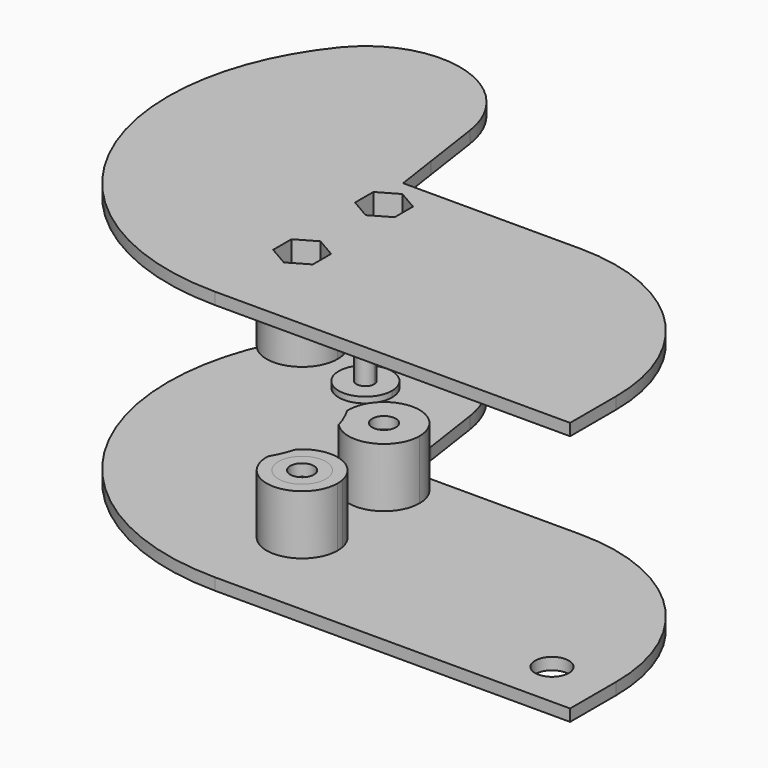
from build123d import *
from build123d import SkipClean  # not in build123d's __all__

# Parameters (mm, degrees)
F0_R      = 4
F1_DEPTH  = 2
F2_DEPTH  = 1
F3_DEPTH  = 10
F4_DEPTH  = 10
F5_R      = 4
F5_R_2    = 2
F6_DEPTH  = 2
F9_DEPTH  = 2
F10_DEPTH = 12
F11_R     = 6
F11_R_2   = 2
F12_DEPTH = 2
F13_DEPTH = 12
F14_R     = 30
F14_2_R   = 30
F15_R     = 2.85
F16_DEPTH = 2


# Not quite as in the source:
# - a feature names something its author has since deleted; it is built from what else it names


with BuildPart() as f1:
    # F0 (on Top) → F1 (new body)
    with BuildSketch(Plane.XY):
        with BuildLine():
            Line((58.100134976, 15), (42.100134976, 15))
            ThreePointArc((42.100134976, 15), (37.6910148186, 1.2250837024), (26.1026494547, -7.4293052282))
            ThreePointArc((26.1026494547, -7.4293052282), (26.1966821755, -8.0364360902), (26.2281363452, -8.65))
            ThreePointArc((26.2281363452, -8.65), (20.0819711782, -14.6482193811), (14.2352577639, -8.3577564209))
            ThreePointArc((14.2352577639, -8.3577564209), (14.2313656207, -8.3570657963), (14.2274735926, -8.3563745231))
            ThreePointArc((14.2274735926, -8.3563745231), (3.8773806963, -16.0379524546), (-8.8387484709, -13.9329295365))
            ThreePointArc((-8.8387484709, -13.9329295365), (3.7392709335, -21.9265497331), (18.3778670292, -24.7222679468))
            ThreePointArc((18.3778670292, -24.7222679468), (46.4657520585, -13.0878850293), (58.100134976, 15))
        make_face()
        with BuildLine():
            ThreePointArc((26.1026494547, -7.4293052282), (37.6910148186, 1.2250837024), (42.100134976, 15))
            Line((42.100134976, 15), (18.3778670292, 15))
            Line((18.3778670292, 15), (11.6619037897, 15))
            ThreePointArc((11.6619037897, 15), (10.5853788563, 14.2218583328), (9.4571172126, 13.5208333333))
            ThreePointArc((9.4571172126, 13.5208333333), (12.1263112553, 11.1893956646), (14.2360603918, 8.3417375001))
            ThreePointArc((14.2360603918, 8.3417375001), (20.0739541807, 14.6480186612), (26.2281363452, 8.65))
            ThreePointArc((26.2281363452, 8.65), (22.4446837804, 3.0744356817), (15.8658305227, 4.5304990701))
            ThreePointArc((15.8658305227, 4.5304990701), (16.3406885354, 2.2873342973), (16.5, 0))
            ThreePointArc((16.5, 0), (16.3406885354, -2.2873342973), (15.8658305227, -4.5304990701))
            ThreePointArc((15.8658305227, -4.5304990701), (21.8629029968, -2.876999221), (26.1026494547, -7.4293052282))
        make_face()
        with BuildLine():
            ThreePointArc((26.2281363452, -8.65), (26.1966821755, -8.0364360902), (26.1026494547, -7.4293052282))
            ThreePointArc((26.1026494547, -7.4293052282), (25.145129633, -7.7365378497), (24.1754492625, -8.0029136587))
            ThreePointArc((24.1754492625, -8.0029136587), (24.2149428159, -8.3253861287), (24.2281363452, -8.65))
            ThreePointArc((24.2281363452, -8.65), (20.2154709299, -12.6499799484), (16.2282165516, -8.6246692964))
            ThreePointArc((16.2282165516, -8.6246692964), (15.2289078696, -8.5123383089), (14.2352577639, -8.3577564209))
            ThreePointArc((14.2352577639, -8.3577564209), (20.0819711782, -14.6482193811), (26.2281363452, -8.65))
        make_face()
        with BuildLine():
            ThreePointArc((24.1754492625, -8.0029136587), (25.145129633, -7.7365378497), (26.1026494547, -7.4293052282))
            ThreePointArc((26.1026494547, -7.4293052282), (21.8629029968, -2.876999221), (15.8658305227, -4.5304990701))
            ThreePointArc((15.8658305227, -4.5304990701), (15.1711022589, -6.4875), (14.2360603918, -8.3417375001))
            ThreePointArc((14.2360603918, -8.3417375001), (14.2356537252, -8.3497466923), (14.2352577639, -8.3577564209))
            ThreePointArc((14.2352577639, -8.3577564209), (15.2289078696, -8.5123383089), (16.2282165516, -8.6246692964))
            ThreePointArc((16.2282165516, -8.6246692964), (19.916147741, -4.6621856725), (24.1754492625, -8.0029136587))
        make_face()
        with BuildLine():
            Line((11.6619037897, 15), (18.3778670292, 15))
            Line((18.3778670292, 15), (17.3205716767, 22.1898913713))
            ThreePointArc((17.3205716767, 22.1898913713), (14.9304924742, 18.2492385576), (11.6619037897, 15))
        make_face()
        with BuildLine():
            Line((78.3778670292, 15), (58.100134976, 15))
            ThreePointArc((58.100134976, 15), (46.4657520585, -13.0878850293), (18.3778670292, -24.7222679468))
            Line((18.3778670292, -24.7222679468), (78.3778670292, -24.7222679468))
            Line((78.3778670292, -24.7222679468), (78.3778670292, 15))
        make_face()
        with BuildLine():
            ThreePointArc((14.2360603918, -8.3417375001), (14.7113718874, -6.2909090909), (15.8658305227, -4.5304990701))
            ThreePointArc((15.8658305227, -4.5304990701), (16.3406885354, -2.2873342973), (16.5, 0))
            ThreePointArc((16.5, 0), (16.3406885354, 2.2873342973), (15.8658305227, 4.5304990701))
            ThreePointArc((15.8658305227, 4.5304990701), (14.7113718874, 6.2909090909), (14.2360603918, 8.3417375001))
            ThreePointArc((14.2360603918, 8.3417375001), (12.1263112553, 11.1893956646), (9.4571172126, 13.5208333333))
            ThreePointArc((9.4571172126, 13.5208333333), (2.354500942, 11.1464505911), (-5.113909886, 11.7011496077))
            ThreePointArc((-5.113909886, 11.7011496077), (1.3016126389, -1.4665580052), (14.2274735926, -8.3563745231))
            ThreePointArc((14.2274735926, -8.3563745231), (14.231768874, -8.3490571155), (14.2360603918, -8.3417375001))
        make_face()
        with BuildLine():
            ThreePointArc((14.2360603918, -8.3417375001), (15.1711022589, -6.4875), (15.8658305227, -4.5304990701))
            ThreePointArc((15.8658305227, -4.5304990701), (14.7113718874, -6.2909090909), (14.2360603918, -8.3417375001))
        make_face()
        with BuildLine():
            Line((6.8738635424, 15), (11.6619037897, 15))
            ThreePointArc((11.6619037897, 15), (14.9304924742, 18.2492385576), (17.3205716767, 22.1898913713))
            Line((17.3205716767, 22.1898913713), (15.8297593001, 32.3278145331))
            ThreePointArc((15.8297593001, 32.3278145331), (15.9573830687, 31.1670156808), (16, 30))
            ThreePointArc((16, 30), (13.3414037895, 21.1678459634), (6.2491318842, 15.2708333333))
            ThreePointArc((6.2491318842, 15.2708333333), (6.562894934, 15.1386396379), (6.8738635424, 15))
        make_face()
        with BuildLine():
            ThreePointArc((9.4571172126, 13.5208333333), (10.5853788563, 14.2218583328), (11.6619037897, 15))
            Line((11.6619037897, 15), (6.8738635424, 15))
            ThreePointArc((6.8738635424, 15), (8.1989155754, 14.3187912684), (9.4571172126, 13.5208333333))
        make_face()
        with BuildLine():
            ThreePointArc((15.8297593001, 32.3278145331), (15.0618472395, 35.3982180146), (13.7045776595, 38.2573937278))
            ThreePointArc((13.7045776595, 38.2573937278), (8.1175093349, 36.3885730362), (3.1632570293, 33.2005944709))
            ThreePointArc((3.1632570293, 33.2005944709), (4.1523882665, 31.734264018), (4.5, 30))
            ThreePointArc((4.5, 30), (2.1202896476, 26.0308222753), (-2.5019430268, 26.2596415826))
            ThreePointArc((-2.5019430268, 26.2596415826), (-4.5458381145, 21.1032564281), (-5.3364742263, 15.6132009157))
            ThreePointArc((-5.3364742263, 15.6132009157), (0.4873806423, 16.4928002507), (6.2491318842, 15.2708333333))
            ThreePointArc((6.2491318842, 15.2708333333), (13.3414037895, 21.1678459634), (16, 30))
            ThreePointArc((16, 30), (15.9573830687, 31.1670156808), (15.8297593001, 32.3278145331))
        make_face()
        with BuildLine():
            ThreePointArc((3.1632570293, 33.2005944709), (8.1175093349, 36.3885730362), (13.7045776595, 38.2573937278))
            ThreePointArc((13.7045776595, 38.2573937278), (1.1371555726, 45.9595387529), (-12.395352396, 40.1170766025))
            ThreePointArc((-12.395352396, 40.1170766025), (-15.5318430865, 26.1578846536), (-6.2491318842, 15.2708333333))
            ThreePointArc((-6.2491318842, 15.2708333333), (-5.7953318392, 15.4487581661), (-5.3364742263, 15.6132009157))
            ThreePointArc((-5.3364742263, 15.6132009157), (-4.5458381145, 21.1032564281), (-2.5019430268, 26.2596415826))
            ThreePointArc((-2.5019430268, 26.2596415826), (-3.4861928807, 32.8454277707), (3.1632570293, 33.2005944709))
        make_face()
        with BuildLine():
            ThreePointArc((-5.113909886, 11.7011496077), (2.354500942, 11.1464505911), (9.4571172126, 13.5208333333))
            ThreePointArc((9.4571172126, 13.5208333333), (8.1989155754, 14.3187912684), (6.8738635424, 15))
            Line((6.8738635424, 15), (5.5677643628, 15))
            ThreePointArc((5.5677643628, 15), (0.1188765047, 14.0004416193), (-5.3442623691, 14.9189237874))
            ThreePointArc((-5.3442623691, 14.9189237874), (-5.2838479343, 13.3061164355), (-5.113909886, 11.7011496077))
        make_face()
        with BuildLine():
            Line((5.5677643628, 15), (6.8738635424, 15))
            ThreePointArc((6.8738635424, 15), (6.562894934, 15.1386396379), (6.2491318842, 15.2708333333))
            ThreePointArc((6.2491318842, 15.2708333333), (5.9099997379, 15.1315130865), (5.5677643628, 15))
        make_face()
        with BuildLine():
            ThreePointArc((-15.4212723827, -5.8680795919), (-12.3953524648, -10.1170765181), (-8.8387484709, -13.9329295365))
            ThreePointArc((-8.8387484709, -13.9329295365), (3.8773806963, -16.0379524546), (14.2274735926, -8.3563745231))
            ThreePointArc((14.2274735926, -8.3563745231), (1.3016126389, -1.4665580052), (-5.113909886, 11.7011496077))
            ThreePointArc((-5.113909886, 11.7011496077), (-7.3421059576, 12.4759171393), (-9.4571172126, 13.5208333333))
            ThreePointArc((-9.4571172126, 13.5208333333), (-15.7707340768, 4.8511799266), (-15.4212723827, -5.8680795919))
        make_face()
        with BuildLine():
            ThreePointArc((4.5, 30), (4.1523882665, 31.734264018), (3.1632570293, 33.2005944709))
            ThreePointArc((3.1632570293, 33.2005944709), (2.0412089663, 32.2005697545), (0.9847414412, 31.1314964843))
            ThreePointArc((0.9847414412, 31.1314964843), (1.3651212697, 30.6216461366), (1.5, 30))
            ThreePointArc((1.5, 30), (0.6644948603, 28.655215043), (-0.9112621076, 28.8085297439))
            ThreePointArc((-0.9112621076, 28.8085297439), (-1.7469963662, 27.5592941625), (-2.5019430268, 26.2596415826))
            ThreePointArc((-2.5019430268, 26.2596415826), (2.1202896476, 26.0308222753), (4.5, 30))
        make_face()
        with BuildLine():
            ThreePointArc((0.9847414412, 31.1314964843), (2.0412089663, 32.2005697545), (3.1632570293, 33.2005944709))
            ThreePointArc((3.1632570293, 33.2005944709), (-3.4861928807, 32.8454277707), (-2.5019430268, 26.2596415826))
            ThreePointArc((-2.5019430268, 26.2596415826), (-1.7469963662, 27.5592941625), (-0.9112621076, 28.8085297439))
            ThreePointArc((-0.9112621076, 28.8085297439), (-1.1620642936, 30.9484759236), (0.9847414412, 31.1314964843))
        make_face()
        with BuildLine():
            ThreePointArc((-6.2491318842, 15.2708333333), (-15.5318430865, 26.1578846536), (-12.395352396, 40.1170766025))
            ThreePointArc((-12.395352396, 40.1170766025), (-16.1558630014, 34.6285521886), (-18.9475622454, 28.5893671785))
            ThreePointArc((-18.9475622454, 28.5893671785), (-16.745225523, 21.0223932931), (-11.6619037897, 15))
            Line((-11.6619037897, 15), (-6.8738635424, 15))
            ThreePointArc((-6.8738635424, 15), (-6.562894934, 15.1386396379), (-6.2491318842, 15.2708333333))
        make_face()
        with BuildLine():
            ThreePointArc((-11.6619037897, 15), (-16.745225523, 21.0223932931), (-18.9475622454, 28.5893671785))
            ThreePointArc((-18.9475622454, 28.5893671785), (-20.7406022259, 21.8995604195), (-21.3444009177, 15))
            Line((-21.3444009177, 15), (-11.6619037897, 15))
        make_face()
        with BuildLine():
            ThreePointArc((14.2360603918, 8.3417375001), (14.7113718874, 6.2909090909), (15.8658305227, 4.5304990701))
            ThreePointArc((15.8658305227, 4.5304990701), (15.1711022589, 6.4875), (14.2360603918, 8.3417375001))
        make_face()
        with BuildLine():
            ThreePointArc((14.2360603918, 8.3417375001), (15.1711022589, 6.4875), (15.8658305227, 4.5304990701))
            ThreePointArc((15.8658305227, 4.5304990701), (22.4446837804, 3.0744356817), (26.2281363452, 8.65))
            ThreePointArc((26.2281363452, 8.65), (20.0739541807, 14.6480186612), (14.2360603918, 8.3417375001))
        make_face()
        with Locations((20.2281363452, 8.65)):
            Circle(F0_R, mode=Mode.SUBTRACT)
        with BuildLine():
            ThreePointArc((-9.4571172126, 13.5208333333), (-7.3421059576, 12.4759171393), (-5.113909886, 11.7011496077))
            ThreePointArc((-5.113909886, 11.7011496077), (-5.2838479343, 13.3061164355), (-5.3442623691, 14.9189237874))
            ThreePointArc((-5.3442623691, 14.9189237874), (-5.4561639627, 14.9590467452), (-5.5677643628, 15))
            Line((-5.5677643628, 15), (-6.8738635424, 15))
            ThreePointArc((-6.8738635424, 15), (-8.1989155754, 14.3187912684), (-9.4571172126, 13.5208333333))
        make_face()
        with BuildLine():
            ThreePointArc((5.5677643628, 15), (5.9099997379, 15.1315130865), (6.2491318842, 15.2708333333))
            ThreePointArc((6.2491318842, 15.2708333333), (0.4873806423, 16.4928002507), (-5.3364742263, 15.6132009157))
            ThreePointArc((-5.3364742263, 15.6132009157), (-5.342419162, 15.3066260733), (-5.3444009177, 15))
            Line((-5.3444009177, 15), (5.5677643628, 15))
        make_face()
        with BuildLine():
            ThreePointArc((-5.3442623691, 14.9189237874), (0.1188765047, 14.0004416193), (5.5677643628, 15))
            Line((5.5677643628, 15), (-5.3444009177, 15))
            ThreePointArc((-5.3444009177, 15), (-5.3443662805, 14.9594618345), (-5.3442623691, 14.9189237874))
        make_face()
        with BuildLine():
            ThreePointArc((-21.3444009177, 15), (-19.834938697, 4.1538002335), (-15.4212723827, -5.8680795919))
            ThreePointArc((-15.4212723827, -5.8680795919), (-15.7707340768, 4.8511799266), (-9.4571172126, 13.5208333333))
            ThreePointArc((-9.4571172126, 13.5208333333), (-10.5853788563, 14.2218583328), (-11.6619037897, 15))
            Line((-11.6619037897, 15), (-21.3444009177, 15))
        make_face()
        with BuildLine():
            ThreePointArc((-5.5677643628, 15), (-5.9099997379, 15.1315130865), (-6.2491318842, 15.2708333333))
            ThreePointArc((-6.2491318842, 15.2708333333), (-6.562894934, 15.1386396379), (-6.8738635424, 15))
            Line((-6.8738635424, 15), (-5.5677643628, 15))
        make_face()
        with BuildLine():
            ThreePointArc((-5.3364742263, 15.6132009157), (-5.7953318392, 15.4487581661), (-6.2491318842, 15.2708333333))
            ThreePointArc((-6.2491318842, 15.2708333333), (-5.9099997379, 15.1315130865), (-5.5677643628, 15))
            Line((-5.5677643628, 15), (-5.3444009177, 15))
            ThreePointArc((-5.3444009177, 15), (-5.342419162, 15.3066260733), (-5.3364742263, 15.6132009157))
        make_face()
        with BuildLine():
            Line((-6.8738635424, 15), (-11.6619037897, 15))
            ThreePointArc((-11.6619037897, 15), (-10.5853788563, 14.2218583328), (-9.4571172126, 13.5208333333))
            ThreePointArc((-9.4571172126, 13.5208333333), (-8.1989155754, 14.3187912684), (-6.8738635424, 15))
        make_face()
        with BuildLine():
            ThreePointArc((-5.5677643628, 15), (-5.4561639627, 14.9590467452), (-5.3442623691, 14.9189237874))
            ThreePointArc((-5.3442623691, 14.9189237874), (-5.3443662805, 14.9594618345), (-5.3444009177, 15))
            Line((-5.3444009177, 15), (-5.5677643628, 15))
        make_face()
    extrude(amount=-F1_DEPTH)

    # F0 (on Top) → F2 (join)
    with BuildSketch(Plane.XY):
        with BuildLine():
            ThreePointArc((4.5, 30), (4.1523882665, 31.734264018), (3.1632570293, 33.2005944709))
            ThreePointArc((3.1632570293, 33.2005944709), (2.0412089663, 32.2005697545), (0.9847414412, 31.1314964843))
            ThreePointArc((0.9847414412, 31.1314964843), (1.3651212697, 30.6216461366), (1.5, 30))
            ThreePointArc((1.5, 30), (0.6644948603, 28.655215043), (-0.9112621076, 28.8085297439))
            ThreePointArc((-0.9112621076, 28.8085297439), (-1.7469963662, 27.5592941625), (-2.5019430268, 26.2596415826))
            ThreePointArc((-2.5019430268, 26.2596415826), (2.1202896476, 26.0308222753), (4.5, 30))
        make_face()
        with BuildLine():
            ThreePointArc((0.9847414412, 31.1314964843), (2.0412089663, 32.2005697545), (3.1632570293, 33.2005944709))
            ThreePointArc((3.1632570293, 33.2005944709), (-3.4861928807, 32.8454277707), (-2.5019430268, 26.2596415826))
            ThreePointArc((-2.5019430268, 26.2596415826), (-1.7469963662, 27.5592941625), (-0.9112621076, 28.8085297439))
            ThreePointArc((-0.9112621076, 28.8085297439), (-1.1620642936, 30.9484759236), (0.9847414412, 31.1314964843))
        make_face()
    with SkipClean():  # cleaning this boolean's faces spoils the solid; the shape is the same uncleaned
        extrude(amount=F2_DEPTH)

    # F0 (on Top) → F3 (join)
    with BuildSketch(Plane.XY):
        with BuildLine():
            ThreePointArc((1.5, 30), (1.3651212697, 30.6216461366), (0.9847414412, 31.1314964843))
            ThreePointArc((0.9847414412, 31.1314964843), (0, 30), (-0.9112621076, 28.8085297439))
            ThreePointArc((-0.9112621076, 28.8085297439), (0.6644948603, 28.655215043), (1.5, 30))
        make_face()
        with BuildLine():
            ThreePointArc((-0.9112621076, 28.8085297439), (0, 30), (0.9847414412, 31.1314964843))
            ThreePointArc((0.9847414412, 31.1314964843), (-1.1620642936, 30.9484759236), (-0.9112621076, 28.8085297439))
        make_face()
    extrude(amount=F3_DEPTH)

    # F0 (on Top) → F4 (join)
    with BuildSketch(Plane.XY):
        with BuildLine():
            ThreePointArc((26.2281363452, -8.65), (26.1966821755, -8.0364360902), (26.1026494547, -7.4293052282))
            ThreePointArc((26.1026494547, -7.4293052282), (25.145129633, -7.7365378497), (24.1754492625, -8.0029136587))
            ThreePointArc((24.1754492625, -8.0029136587), (24.2149428159, -8.3253861287), (24.2281363452, -8.65))
            ThreePointArc((24.2281363452, -8.65), (20.2154709299, -12.6499799484), (16.2282165516, -8.6246692964))
            ThreePointArc((16.2282165516, -8.6246692964), (15.2289078696, -8.5123383089), (14.2352577639, -8.3577564209))
            ThreePointArc((14.2352577639, -8.3577564209), (20.0819711782, -14.6482193811), (26.2281363452, -8.65))
        make_face()
        with BuildLine():
            ThreePointArc((14.2360603918, 8.3417375001), (15.1711022589, 6.4875), (15.8658305227, 4.5304990701))
            ThreePointArc((15.8658305227, 4.5304990701), (22.4446837804, 3.0744356817), (26.2281363452, 8.65))
            ThreePointArc((26.2281363452, 8.65), (20.0739541807, 14.6480186612), (14.2360603918, 8.3417375001))
        make_face()
        with Locations((20.2281363452, 8.65)):
            Circle(F0_R, mode=Mode.SUBTRACT)
        with BuildLine():
            ThreePointArc((24.1754492625, -8.0029136587), (25.145129633, -7.7365378497), (26.1026494547, -7.4293052282))
            ThreePointArc((26.1026494547, -7.4293052282), (21.8629029968, -2.876999221), (15.8658305227, -4.5304990701))
            ThreePointArc((15.8658305227, -4.5304990701), (15.1711022589, -6.4875), (14.2360603918, -8.3417375001))
            ThreePointArc((14.2360603918, -8.3417375001), (14.2356537252, -8.3497466923), (14.2352577639, -8.3577564209))
            ThreePointArc((14.2352577639, -8.3577564209), (15.2289078696, -8.5123383089), (16.2282165516, -8.6246692964))
            ThreePointArc((16.2282165516, -8.6246692964), (19.916147741, -4.6621856725), (24.1754492625, -8.0029136587))
        make_face()
    extrude(amount=F4_DEPTH)

    # F5 (on face) → F6 (join)
    with BuildSketch(Plane.XY.offset(10)):
        with Locations((20.2281363452, 8.65)):
            Circle(F5_R)
        with Locations((20.2281363452, 8.65)):
            Circle(F5_R_2, mode=Mode.SUBTRACT)
        with Locations((20.2281363452, -8.65)):
            Circle(F5_R)
        with Locations((20.2281363452, -8.65)):
            Circle(F5_R_2, mode=Mode.SUBTRACT)
    extrude(amount=-F6_DEPTH)

    # F14
    f14_edges = [f1.edges().sort_by_distance(p)[0] for p in [
        (78.377867, 15, -1),
    ]]
    fillet(f14_edges, radius=F14_R)

    # F15 (on face) → F16 (cut, through all)
    with BuildSketch(Plane(origin=(0, 0, -2), x_dir=(1, 0, 0), z_dir=(0, 0, -1))):
        with Locations((69.0778670292, 16.9222679468)):
            Circle(F15_R)
    extrude(amount=-F16_DEPTH, mode=Mode.SUBTRACT)


with BuildPart() as f9:
    # F8 (on offset) → F9 (new body)
    with BuildSketch(Plane.XY.offset(40.5)):
        with BuildLine():
            Line((58.100134976, 15), (42.100134976, 15))
            ThreePointArc((42.100134976, 15), (37.6910148186, 1.2250837024), (26.1026494547, -7.4293052282))
            ThreePointArc((26.1026494547, -7.4293052282), (26.1966821755, -8.0364360902), (26.2281363452, -8.65))
            ThreePointArc((26.2281363452, -8.65), (20.0819711782, -14.6482193811), (14.2352577639, -8.3577564209))
            ThreePointArc((14.2352577639, -8.3577564209), (14.2313656207, -8.3570657963), (14.2274735926, -8.3563745231))
            ThreePointArc((14.2274735926, -8.3563745231), (3.8773806963, -16.0379524546), (-8.8387484709, -13.9329295365))
            ThreePointArc((-8.8387484709, -13.9329295365), (3.7392709335, -21.9265497331), (18.3778670292, -24.7222679468))
            ThreePointArc((18.3778670292, -24.7222679468), (46.4657520585, -13.0878850293), (58.100134976, 15))
        make_face()
        with BuildLine():
            ThreePointArc((26.1026494547, -7.4293052282), (37.6910148186, 1.2250837024), (42.100134976, 15))
            Line((42.100134976, 15), (18.3778670292, 15))
            Line((18.3778670292, 15), (11.6619037897, 15))
            ThreePointArc((11.6619037897, 15), (10.5853788563, 14.2218583328), (9.4571172126, 13.5208333333))
            ThreePointArc((9.4571172126, 13.5208333333), (12.1263112553, 11.1893956646), (14.2360603918, 8.3417375001))
            ThreePointArc((14.2360603918, 8.3417375001), (20.0739541807, 14.6480186612), (26.2281363452, 8.65))
            ThreePointArc((26.2281363452, 8.65), (22.4446837804, 3.0744356817), (15.8658305227, 4.5304990701))
            ThreePointArc((15.8658305227, 4.5304990701), (16.3406885354, 2.2873342973), (16.5, 0))
            ThreePointArc((16.5, 0), (16.3406885354, -2.2873342973), (15.8658305227, -4.5304990701))
            ThreePointArc((15.8658305227, -4.5304990701), (21.8629029968, -2.876999221), (26.1026494547, -7.4293052282))
        make_face()
        with BuildLine():
            ThreePointArc((26.2281363452, -8.65), (26.1966821755, -8.0364360902), (26.1026494547, -7.4293052282))
            ThreePointArc((26.1026494547, -7.4293052282), (24.8503000713, -7.8222174001), (23.5781363452, -8.1452629188))
            Line((23.5781363452, -8.1452629188), (23.5781363452, -10.5841234018))
            Line((23.5781363452, -10.5841234018), (20.2281363452, -12.5182468036))
            Line((20.2281363452, -12.5182468036), (16.8781363452, -10.5841234018))
            Line((16.8781363452, -10.5841234018), (16.8781363452, -8.6748137145))
            ThreePointArc((16.8781363452, -8.6748137145), (15.5522465031, -8.5533833065), (14.2352577639, -8.3577564209))
            ThreePointArc((14.2352577639, -8.3577564209), (20.0819711782, -14.6482193811), (26.2281363452, -8.65))
        make_face()
        with BuildLine():
            ThreePointArc((23.5781363452, -8.1452629188), (24.8503000713, -7.8222174001), (26.1026494547, -7.4293052282))
            ThreePointArc((26.1026494547, -7.4293052282), (21.8629029968, -2.876999221), (15.8658305227, -4.5304990701))
            ThreePointArc((15.8658305227, -4.5304990701), (15.1711022589, -6.4875), (14.2360603918, -8.3417375001))
            ThreePointArc((14.2360603918, -8.3417375001), (14.2356537252, -8.3497466923), (14.2352577639, -8.3577564209))
            ThreePointArc((14.2352577639, -8.3577564209), (15.5522465031, -8.5533833065), (16.8781363452, -8.6748137145))
            Line((16.8781363452, -8.6748137145), (16.8781363452, -6.7158765982))
            Line((16.8781363452, -6.7158765982), (20.2281363452, -4.7817531964))
            Line((20.2281363452, -4.7817531964), (23.5781363452, -6.7158765982))
            Line((23.5781363452, -6.7158765982), (23.5781363452, -8.1452629188))
        make_face()
        with BuildLine():
            Line((11.6619037897, 15), (18.3778670292, 15))
            Line((18.3778670292, 15), (17.3205716767, 22.1898913713))
            ThreePointArc((17.3205716767, 22.1898913713), (14.9304924742, 18.2492385576), (11.6619037897, 15))
        make_face()
        with BuildLine():
            Line((78.3778670292, 15), (58.100134976, 15))
            ThreePointArc((58.100134976, 15), (46.4657520585, -13.0878850293), (18.3778670292, -24.7222679468))
            Line((18.3778670292, -24.7222679468), (78.3778670292, -24.7222679468))
            Line((78.3778670292, -24.7222679468), (78.3778670292, 15))
        make_face()
        with BuildLine():
            ThreePointArc((14.2360603918, -8.3417375001), (14.7113718874, -6.2909090909), (15.8658305227, -4.5304990701))
            ThreePointArc((15.8658305227, -4.5304990701), (16.3406885354, -2.2873342973), (16.5, 0))
            ThreePointArc((16.5, 0), (16.3406885354, 2.2873342973), (15.8658305227, 4.5304990701))
            ThreePointArc((15.8658305227, 4.5304990701), (14.7113718874, 6.2909090909), (14.2360603918, 8.3417375001))
            ThreePointArc((14.2360603918, 8.3417375001), (12.1263112553, 11.1893956646), (9.4571172126, 13.5208333333))
            ThreePointArc((9.4571172126, 13.5208333333), (2.354500942, 11.1464505911), (-5.113909886, 11.7011496077))
            ThreePointArc((-5.113909886, 11.7011496077), (1.3016126389, -1.4665580052), (14.2274735926, -8.3563745231))
            ThreePointArc((14.2274735926, -8.3563745231), (14.231768874, -8.3490571155), (14.2360603918, -8.3417375001))
        make_face()
        with BuildLine():
            ThreePointArc((14.2360603918, -8.3417375001), (15.1711022589, -6.4875), (15.8658305227, -4.5304990701))
            ThreePointArc((15.8658305227, -4.5304990701), (14.7113718874, -6.2909090909), (14.2360603918, -8.3417375001))
        make_face()
        with BuildLine():
            Line((6.8738635424, 15), (11.6619037897, 15))
            ThreePointArc((11.6619037897, 15), (14.9304924742, 18.2492385576), (17.3205716767, 22.1898913713))
            Line((17.3205716767, 22.1898913713), (15.8297593556, 32.3278141558))
            ThreePointArc((15.8297593556, 32.3278141558), (15.9573830826, 31.1670154906), (16, 30))
            ThreePointArc((16, 30), (13.3414037895, 21.1678459634), (6.2491318842, 15.2708333333))
            ThreePointArc((6.2491318842, 15.2708333333), (6.562894934, 15.1386396379), (6.8738635424, 15))
        make_face()
        with BuildLine():
            ThreePointArc((9.4571172126, 13.5208333333), (10.5853788563, 14.2218583328), (11.6619037897, 15))
            Line((11.6619037897, 15), (6.8738635424, 15))
            ThreePointArc((6.8738635424, 15), (8.1989155754, 14.3187912684), (9.4571172126, 13.5208333333))
        make_face()
        with BuildLine():
            ThreePointArc((15.8297593556, 32.3278141558), (15.0618473039, 35.3982178351), (13.7045776595, 38.2573937278))
            ThreePointArc((13.7045776595, 38.2573937278), (7.8917709447, 36.2788107151), (2.781523926, 32.8745651234))
            ThreePointArc((2.781523926, 32.8745651234), (3.6828043462, 31.5610740366), (4, 30))
            ThreePointArc((4, 30), (1.8660095282, 26.4619202326), (-2.2590042204, 26.6989547213))
            ThreePointArc((-2.2590042204, 26.6989547213), (-4.4799761986, 21.3454707876), (-5.3364742263, 15.6132009157))
            ThreePointArc((-5.3364742263, 15.6132009157), (0.4873806423, 16.4928002507), (6.2491318842, 15.2708333333))
            ThreePointArc((6.2491318842, 15.2708333333), (13.3414037895, 21.1678459634), (16, 30))
            ThreePointArc((16, 30), (15.9573830826, 31.1670154906), (15.8297593556, 32.3278141558))
        make_face()
        with BuildLine():
            ThreePointArc((2.781523926, 32.8745651234), (7.8917709447, 36.2788107151), (13.7045776595, 38.2573937278))
            ThreePointArc((13.7045776595, 38.2573937278), (1.1371555726, 45.9595387529), (-12.395352396, 40.1170766025))
            ThreePointArc((-12.395352396, 40.1170766025), (-15.5318430865, 26.1578846536), (-6.2491318842, 15.2708333333))
            ThreePointArc((-6.2491318842, 15.2708333333), (-5.7953318392, 15.4487581661), (-5.3364742263, 15.6132009157))
            ThreePointArc((-5.3364742263, 15.6132009157), (-4.4799761986, 21.3454707876), (-2.2590042204, 26.6989547213))
            ThreePointArc((-2.2590042204, 26.6989547213), (-3.0988381162, 32.5292691295), (2.781523926, 32.8745651234))
        make_face()
        with BuildLine():
            ThreePointArc((14.2274735926, -8.3563745231), (14.2313656207, -8.3570657963), (14.2352577639, -8.3577564209))
            ThreePointArc((14.2352577639, -8.3577564209), (14.2356537252, -8.3497466923), (14.2360603918, -8.3417375001))
            ThreePointArc((14.2360603918, -8.3417375001), (14.231768874, -8.3490571155), (14.2274735926, -8.3563745231))
        make_face()
        with BuildLine():
            ThreePointArc((-5.113909886, 11.7011496077), (2.354500942, 11.1464505911), (9.4571172126, 13.5208333333))
            ThreePointArc((9.4571172126, 13.5208333333), (8.1989155754, 14.3187912684), (6.8738635424, 15))
            Line((6.8738635424, 15), (5.5677643628, 15))
            ThreePointArc((5.5677643628, 15), (0.1188765047, 14.0004416193), (-5.3442623691, 14.9189237874))
            ThreePointArc((-5.3442623691, 14.9189237874), (-5.2838479343, 13.3061164355), (-5.113909886, 11.7011496077))
        make_face()
        with BuildLine():
            Line((5.5677643628, 15), (6.8738635424, 15))
            ThreePointArc((6.8738635424, 15), (6.562894934, 15.1386396379), (6.2491318842, 15.2708333333))
            ThreePointArc((6.2491318842, 15.2708333333), (5.9099997379, 15.1315130865), (5.5677643628, 15))
        make_face()
        with BuildLine():
            ThreePointArc((-15.4212723827, -5.8680795919), (-12.3953524648, -10.1170765181), (-8.8387484709, -13.9329295365))
            ThreePointArc((-8.8387484709, -13.9329295365), (3.8773806963, -16.0379524546), (14.2274735926, -8.3563745231))
            ThreePointArc((14.2274735926, -8.3563745231), (1.3016126389, -1.4665580052), (-5.113909886, 11.7011496077))
            ThreePointArc((-5.113909886, 11.7011496077), (-7.3421059576, 12.4759171393), (-9.4571172126, 13.5208333333))
            ThreePointArc((-9.4571172126, 13.5208333333), (-15.7707340768, 4.8511799266), (-15.4212723827, -5.8680795919))
        make_face()
        with BuildLine():
            ThreePointArc((4, 30), (3.6828043462, 31.5610740366), (2.781523926, 32.8745651234))
            ThreePointArc((2.781523926, 32.8745651234), (2.0406007003, 32.1999920186), (1.3288254001, 31.4947317672))
            ThreePointArc((1.3288254001, 31.4947317672), (1.8245068923, 30.8192524641), (2, 30))
            ThreePointArc((2, 30), (0.8954353836, 28.2116500696), (-1.1981954737, 28.3986481939))
            ThreePointArc((-1.1981954737, 28.3986481939), (-1.7465522102, 27.5600058448), (-2.2590042204, 26.6989547213))
            ThreePointArc((-2.2590042204, 26.6989547213), (1.8660095282, 26.4619202326), (4, 30))
        make_face()
        with BuildLine():
            ThreePointArc((1.3288254001, 31.4947317672), (2.0406007003, 32.1999920186), (2.781523926, 32.8745651234))
            ThreePointArc((2.781523926, 32.8745651234), (-3.0988381162, 32.5292691295), (-2.2590042204, 26.6989547213))
            ThreePointArc((-2.2590042204, 26.6989547213), (-1.7465522102, 27.5600058448), (-1.1981954737, 28.3986481939))
            ThreePointArc((-1.1981954737, 28.3986481939), (-1.5494190581, 31.2646345648), (1.3288254001, 31.4947317672))
        make_face()
        with BuildLine():
            ThreePointArc((-6.2491318842, 15.2708333333), (-15.5318430865, 26.1578846536), (-12.395352396, 40.1170766025))
            ThreePointArc((-12.395352396, 40.1170766025), (-16.1558630014, 34.6285521886), (-18.9475622454, 28.5893671785))
            ThreePointArc((-18.9475622454, 28.5893671785), (-16.745225523, 21.0223932931), (-11.6619037897, 15))
            Line((-11.6619037897, 15), (-6.8738635424, 15))
            ThreePointArc((-6.8738635424, 15), (-6.562894934, 15.1386396379), (-6.2491318842, 15.2708333333))
        make_face()
        with BuildLine():
            ThreePointArc((-11.6619037897, 15), (-16.745225523, 21.0223932931), (-18.9475622454, 28.5893671785))
            ThreePointArc((-18.9475622454, 28.5893671785), (-20.7406022259, 21.8995604195), (-21.3444009177, 15))
            Line((-21.3444009177, 15), (-11.6619037897, 15))
        make_face()
        with BuildLine():
            ThreePointArc((14.2360603918, 8.3417375001), (14.7113718874, 6.2909090909), (15.8658305227, 4.5304990701))
            ThreePointArc((15.8658305227, 4.5304990701), (15.1711022589, 6.4875), (14.2360603918, 8.3417375001))
        make_face()
        with BuildLine():
            ThreePointArc((14.2360603918, 8.3417375001), (15.1711022589, 6.4875), (15.8658305227, 4.5304990701))
            ThreePointArc((15.8658305227, 4.5304990701), (22.4446837804, 3.0744356817), (26.2281363452, 8.65))
            ThreePointArc((26.2281363452, 8.65), (20.0739541807, 14.6480186612), (14.2360603918, 8.3417375001))
        make_face()
        Polygon((20.2281363452, 12.5182468036), (23.5781363452, 10.5841234018), (23.5781363452, 6.7158765982), (20.2281363452, 4.7817531964), (16.8781363452, 6.7158765982), (16.8781363452, 10.5841234018), align=None, mode=Mode.SUBTRACT)
        with BuildLine():
            ThreePointArc((-9.4571172126, 13.5208333333), (-7.3421059576, 12.4759171393), (-5.113909886, 11.7011496077))
            ThreePointArc((-5.113909886, 11.7011496077), (-5.2838479343, 13.3061164355), (-5.3442623691, 14.9189237874))
            ThreePointArc((-5.3442623691, 14.9189237874), (-5.4561639627, 14.9590467452), (-5.5677643628, 15))
            Line((-5.5677643628, 15), (-6.8738635424, 15))
            ThreePointArc((-6.8738635424, 15), (-8.1989155754, 14.3187912684), (-9.4571172126, 13.5208333333))
        make_face()
        with BuildLine():
            ThreePointArc((5.5677643628, 15), (5.9099997379, 15.1315130865), (6.2491318842, 15.2708333333))
            ThreePointArc((6.2491318842, 15.2708333333), (0.4873806423, 16.4928002507), (-5.3364742263, 15.6132009157))
            ThreePointArc((-5.3364742263, 15.6132009157), (-5.342419162, 15.3066260733), (-5.3444009177, 15))
            Line((-5.3444009177, 15), (5.5677643628, 15))
        make_face()
        with BuildLine():
            ThreePointArc((-5.3442623691, 14.9189237874), (0.1188765047, 14.0004416193), (5.5677643628, 15))
            Line((5.5677643628, 15), (-5.3444009177, 15))
            ThreePointArc((-5.3444009177, 15), (-5.3443662805, 14.9594618345), (-5.3442623691, 14.9189237874))
        make_face()
        with BuildLine():
            ThreePointArc((-21.3444009177, 15), (-19.834938697, 4.1538002335), (-15.4212723827, -5.8680795919))
            ThreePointArc((-15.4212723827, -5.8680795919), (-15.7707340768, 4.8511799266), (-9.4571172126, 13.5208333333))
            ThreePointArc((-9.4571172126, 13.5208333333), (-10.5853788563, 14.2218583328), (-11.6619037897, 15))
            Line((-11.6619037897, 15), (-21.3444009177, 15))
        make_face()
        with BuildLine():
            ThreePointArc((2, 30), (1.8245068923, 30.8192524641), (1.3288254001, 31.4947317672))
            ThreePointArc((1.3288254001, 31.4947317672), (0, 30), (-1.1981954737, 28.3986481939))
            ThreePointArc((-1.1981954737, 28.3986481939), (0.8954353836, 28.2116500696), (2, 30))
        make_face()
        with BuildLine():
            ThreePointArc((-1.1981954737, 28.3986481939), (0, 30), (1.3288254001, 31.4947317672))
            ThreePointArc((1.3288254001, 31.4947317672), (-1.5494190581, 31.2646345648), (-1.1981954737, 28.3986481939))
        make_face()
        with BuildLine():
            ThreePointArc((-5.5677643628, 15), (-5.9099997379, 15.1315130865), (-6.2491318842, 15.2708333333))
            ThreePointArc((-6.2491318842, 15.2708333333), (-6.562894934, 15.1386396379), (-6.8738635424, 15))
            Line((-6.8738635424, 15), (-5.5677643628, 15))
        make_face()
        with BuildLine():
            ThreePointArc((-5.3364742263, 15.6132009157), (-5.7953318392, 15.4487581661), (-6.2491318842, 15.2708333333))
            ThreePointArc((-6.2491318842, 15.2708333333), (-5.9099997379, 15.1315130865), (-5.5677643628, 15))
            Line((-5.5677643628, 15), (-5.3444009177, 15))
            ThreePointArc((-5.3444009177, 15), (-5.342419162, 15.3066260733), (-5.3364742263, 15.6132009157))
        make_face()
        with BuildLine():
            Line((-6.8738635424, 15), (-11.6619037897, 15))
            ThreePointArc((-11.6619037897, 15), (-10.5853788563, 14.2218583328), (-9.4571172126, 13.5208333333))
            ThreePointArc((-9.4571172126, 13.5208333333), (-8.1989155754, 14.3187912684), (-6.8738635424, 15))
        make_face()
        with BuildLine():
            ThreePointArc((-5.5677643628, 15), (-5.4561639627, 14.9590467452), (-5.3442623691, 14.9189237874))
            ThreePointArc((-5.3442623691, 14.9189237874), (-5.3443662805, 14.9594618345), (-5.3444009177, 15))
            Line((-5.3444009177, 15), (-5.5677643628, 15))
        make_face()
    extrude(amount=F9_DEPTH)

    # F8 (on offset) → F10 (join)
    with BuildSketch(Plane.XY.offset(40.5)):
        with BuildLine():
            ThreePointArc((26.2281363452, -8.65), (26.1966821755, -8.0364360902), (26.1026494547, -7.4293052282))
            ThreePointArc((26.1026494547, -7.4293052282), (24.8503000713, -7.8222174001), (23.5781363452, -8.1452629188))
            Line((23.5781363452, -8.1452629188), (23.5781363452, -10.5841234018))
            Line((23.5781363452, -10.5841234018), (20.2281363452, -12.5182468036))
            Line((20.2281363452, -12.5182468036), (16.8781363452, -10.5841234018))
            Line((16.8781363452, -10.5841234018), (16.8781363452, -8.6748137145))
            ThreePointArc((16.8781363452, -8.6748137145), (15.5522465031, -8.5533833065), (14.2352577639, -8.3577564209))
            ThreePointArc((14.2352577639, -8.3577564209), (20.0819711782, -14.6482193811), (26.2281363452, -8.65))
        make_face()
        with BuildLine():
            ThreePointArc((23.5781363452, -8.1452629188), (24.8503000713, -7.8222174001), (26.1026494547, -7.4293052282))
            ThreePointArc((26.1026494547, -7.4293052282), (21.8629029968, -2.876999221), (15.8658305227, -4.5304990701))
            ThreePointArc((15.8658305227, -4.5304990701), (15.1711022589, -6.4875), (14.2360603918, -8.3417375001))
            ThreePointArc((14.2360603918, -8.3417375001), (14.2356537252, -8.3497466923), (14.2352577639, -8.3577564209))
            ThreePointArc((14.2352577639, -8.3577564209), (15.5522465031, -8.5533833065), (16.8781363452, -8.6748137145))
            Line((16.8781363452, -8.6748137145), (16.8781363452, -6.7158765982))
            Line((16.8781363452, -6.7158765982), (20.2281363452, -4.7817531964))
            Line((20.2281363452, -4.7817531964), (23.5781363452, -6.7158765982))
            Line((23.5781363452, -6.7158765982), (23.5781363452, -8.1452629188))
        make_face()
        with BuildLine():
            ThreePointArc((14.2360603918, -8.3417375001), (15.1711022589, -6.4875), (15.8658305227, -4.5304990701))
            ThreePointArc((15.8658305227, -4.5304990701), (14.7113718874, -6.2909090909), (14.2360603918, -8.3417375001))
        make_face()
        with BuildLine():
            ThreePointArc((14.2360603918, 8.3417375001), (14.7113718874, 6.2909090909), (15.8658305227, 4.5304990701))
            ThreePointArc((15.8658305227, 4.5304990701), (15.1711022589, 6.4875), (14.2360603918, 8.3417375001))
        make_face()
        with BuildLine():
            ThreePointArc((14.2360603918, 8.3417375001), (15.1711022589, 6.4875), (15.8658305227, 4.5304990701))
            ThreePointArc((15.8658305227, 4.5304990701), (22.4446837804, 3.0744356817), (26.2281363452, 8.65))
            ThreePointArc((26.2281363452, 8.65), (20.0739541807, 14.6480186612), (14.2360603918, 8.3417375001))
        make_face()
        Polygon((20.2281363452, 12.5182468036), (23.5781363452, 10.5841234018), (23.5781363452, 6.7158765982), (20.2281363452, 4.7817531964), (16.8781363452, 6.7158765982), (16.8781363452, 10.5841234018), align=None, mode=Mode.SUBTRACT)
    extrude(amount=-F10_DEPTH)

    # F11 (on face) → F12 (join)
    with BuildSketch(Plane(origin=(0, 0, 28.5), x_dir=(1, 0, 0), z_dir=(0, 0, -1))):
        with Locations((20.2281363452, 8.65)):
            Circle(F11_R)
        Polygon((16.8781363452, 10.5841234018), (20.2281363452, 12.5182468036), (23.5781363452, 10.5841234018), (23.5781363452, 6.7158765982), (20.2281363452, 4.7817531964), (16.8781363452, 6.7158765982), align=None, mode=Mode.SUBTRACT)
        with Locations((20.2281363452, -8.65)):
            Circle(F11_R)
        with Locations((20.2281363452, -8.65)):
            Circle(F11_R_2, mode=Mode.SUBTRACT)
        Polygon((23.5781363452, 10.5841234018), (20.2281363452, 12.5182468036), (16.8781363452, 10.5841234018), (16.8781363452, 6.7158765982), (20.2281363452, 4.7817531964), (23.5781363452, 6.7158765982), align=None)
        with Locations((20.2281363452, 8.65)):
            Circle(F11_R_2, mode=Mode.SUBTRACT)
    extrude(amount=-F12_DEPTH)

    # F8 (on offset) → F13 (join)
    with BuildSketch(Plane.XY.offset(40.5)):
        with BuildLine():
            ThreePointArc((-1.1981954737, 28.3986481939), (0, 30), (1.3288254001, 31.4947317672))
            ThreePointArc((1.3288254001, 31.4947317672), (-1.5494190581, 31.2646345648), (-1.1981954737, 28.3986481939))
        make_face()
        with BuildLine():
            ThreePointArc((2, 30), (1.8245068923, 30.8192524641), (1.3288254001, 31.4947317672))
            ThreePointArc((1.3288254001, 31.4947317672), (0, 30), (-1.1981954737, 28.3986481939))
            ThreePointArc((-1.1981954737, 28.3986481939), (0.8954353836, 28.2116500696), (2, 30))
        make_face()
    extrude(amount=-F13_DEPTH)

    # F14#2
    f14_2_edges = [f9.edges().sort_by_distance(p)[0] for p in [
        (78.377867, 15, 41.5),
    ]]
    fillet(f14_2_edges, radius=F14_2_R)


solid = Compound([f1.part, f9.part])
